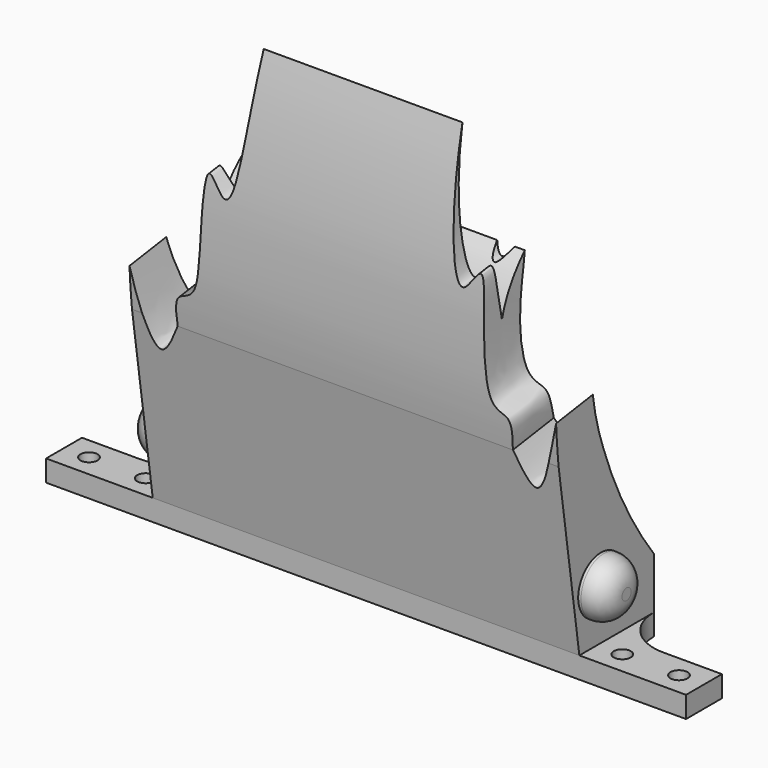
from build123d import *

# Parameters (mm, degrees)
F0_R      = 1.5
F1_DEPTH  = 3.75
F2_W      = 75
F2_H      = 7.89
F3_DEPTH  = 10
F4_W      = 75
F4_H      = 13.75
F5_DEPTH  = 25
F7_DEPTH  = 108.8
F9_DEPTH  = 25
F10_W     = 23.3560199849
F10_H     = 16.445
F11_DEPTH = 5
F15_DEPTH = 75
F17_DEPTH = 25
F19_R     = 8.4497474683
F20_DEPTH = 4
F22_DEPTH = 113.6
F23_R     = 5
F24_DEPTH = 4.5
F25_R     = 4
F26_R     = 5
F27_DEPTH = 4.5
F28_R     = 4


# Not quite as in the source:
# - a feature of the source that left no trace in its solid (it failed there, or was rolled back) is left out


with BuildPart() as f1:
    # F0 (on Top) → F1 (new body)
    with BuildSketch(Plane.XY):
        Polygon((-20.03, 3.5297368421), (-38.78, 3.5297368421), (-38.78, -4.3602631579), (73.72, -4.3602631579), (73.72, 3.5297368421), align=None)
        with Locations((-34.39, -0.4152631579)):
            Circle(F0_R, mode=Mode.SUBTRACT)
        with BuildLine():
            ThreePointArc((-22.92, -0.4152631579), (-24.42, -1.9152631579), (-25.92, -0.4152631579))
            ThreePointArc((-25.92, -0.4152631579), (-24.42, 1.0847368421), (-22.92, -0.4152631579))
        make_face(mode=Mode.SUBTRACT)
        with Locations((-15.64, -0.4152631579)):
            Circle(F0_R, mode=Mode.SUBTRACT)
        with Locations((-5.67, -0.4152631579)):
            Circle(F0_R, mode=Mode.SUBTRACT)
        with Locations((3.11, -0.4152631579)):
            Circle(F0_R, mode=Mode.SUBTRACT)
        with Locations((13.08, -0.4152631579)):
            Circle(F0_R, mode=Mode.SUBTRACT)
        with Locations((21.86, -0.4152631579)):
            Circle(F0_R, mode=Mode.SUBTRACT)
        with Locations((31.83, -0.4152631579)):
            Circle(F0_R, mode=Mode.SUBTRACT)
        with Locations((40.61, -0.4152631579)):
            Circle(F0_R, mode=Mode.SUBTRACT)
        with Locations((50.58, -0.4152631579)):
            Circle(F0_R, mode=Mode.SUBTRACT)
        with Locations((59.36, -0.4152631579)):
            Circle(F0_R, mode=Mode.SUBTRACT)
        with Locations((69.33, -0.4152631579)):
            Circle(F0_R, mode=Mode.SUBTRACT)
    extrude(amount=F1_DEPTH)

    # F2 (on face) → F3 (join)
    with BuildSketch(Plane.XY.offset(3.75)):
        with Locations((17.47, -0.4152631579)):
            Rectangle(F2_W, F2_H)
    extrude(amount=F3_DEPTH)

    # F4 (on face) → F5 (join)
    with BuildSketch(Plane(origin=(0, 3.5297368421, 0), x_dir=(-1, 0, 0), z_dir=(0, 1, 0))):
        with Locations((-17.47, 6.875)):
            Rectangle(F4_W, F4_H)
    extrude(amount=F5_DEPTH)

    # F6 (on face) → F7 (cut)
    with BuildSketch(Plane(origin=(-20.03, 0, 0), x_dir=(0, -1, 0), z_dir=(-1, 0, 0))):
        with BuildLine():
            Line((-28.5297368421, 13.75), (-28.5297368421, 1.3423696908))
            add(Edge.make_bspline(
                [(-28.5297368421, 1.3423696908), (-28.4407085002, 1.8407238057), (-27.4309487298, 4.2160851583), (-18.5019975598, 9.7006212436), (-25.1355636842, 11.5607893027), (-17.452811929, 12.8495323479), (-12.0847368421, 13.75)],
                knots=[0.0902573519, 0.0902573519, 0.0902573519, 0.0902573519, 0.1853961314, 0.5083170397, 0.656452384, 1, 1, 1, 1], degree=3))
            Line((-12.0847368421, 13.75), (-28.5297368421, 13.75))
        make_face()
    extrude(amount=-F7_DEPTH, mode=Mode.SUBTRACT)

    # F8 (on face) → F9 (cut)
    with BuildSketch(Plane.XY.offset(13.75)):
        with BuildLine():
            Line((-20.03, 28.5297368421), (-20.03, 12.0847368421))
            add(Edge.make_bspline(
                [(-20.03, 12.0847368421), (-16.6011347781, 15.620817943), (-11.1074776006, 21.8320831182), (-6.6512433884, 13.3190321336), (-3.164406946, 31.8472349575), (7.0542574353, 21.7542281947), (14.4432723922, 26.9517716178), (17.47, 28.5297368421)],
                knots=[0, 0, 0, 0, 0.2253636629, 0.3548505417, 0.5781774765, 0.7768820918, 1, 1, 1, 1], degree=3))
            Line((17.47, 28.5297368421), (-20.03, 28.5297368421))
        make_face()
        with BuildLine():
            Line((54.97, 28.5297368421), (17.47, 28.5297368421))
            add(Edge.make_bspline(
                [(54.97, 12.0847368421), (51.5411347781, 15.620817943), (46.0474776006, 21.8320831182), (41.5912433884, 13.3190321336), (38.104406946, 31.8472349575), (27.8857425647, 21.7542281947), (20.4967276078, 26.9517716178), (17.47, 28.5297368421)],
                knots=[0, 0, 0, 0, 0.2253636629, 0.3548505417, 0.5781774765, 0.7768820918, 1, 1, 1, 1], degree=3))
            Line((54.97, 12.0847368421), (54.97, 28.5297368421))
        make_face()
    extrude(amount=-F9_DEPTH, mode=Mode.SUBTRACT)

    # F10 (on face) → F11 (join)
    with BuildSketch(Plane.XY.offset(13.75)):
        with Locations((28.7449785974, 3.8622368421)):
            Rectangle(F10_W, F10_H)
        with Locations((5.3889586125, 3.8622368421)):
            Rectangle(F10_W, F10_H)
        Polygon((17.0669686049, 17.9865639657), (17.0669686049, 12.0847368421), (40.4229885899, 12.0847368421), align=None)
        Polygon((17.0669686049, 17.9865639657), (-6.28905138, 12.0847368421), (17.0669686049, 12.0847368421), align=None)
    extrude(amount=F11_DEPTH)

    # F14 (on face) → F15 (join)
    with BuildSketch(Plane(origin=(-20.03, 0, 0), x_dir=(0, -1, 0), z_dir=(-1, 0, 0))):
        with BuildLine():
            Line((4.3602631579, 0), (4.3602631579, 3.75))
            Line((4.3602631579, 3.75), (8.9196669428, 34.7869201625))
            ThreePointArc((8.9196669428, 34.7869201625), (9.1775200626, 57.5848380943), (5.009538897, 80))
            ThreePointArc((5.009538897, 80), (6.7748915404, 66.0775688262), (5.5820018111, 52.0944513684))
            ThreePointArc((5.5820018111, 52.0944513684), (3.0013036661, 42.5791343604), (-0.9565926029, 33.5493880847))
            ThreePointArc((-0.9565926029, 33.5493880847), (-8.0005792846, 22.8777948312), (-16.9551318954, 13.75))
            Line((-16.9551318954, 13.75), (-5.9577007778, 13.75))
            Line((-5.9577007778, 13.75), (-5.9577007778, 0))
            Line((-5.9577007778, 0), (4.3602631579, 0))
        make_face()
        with BuildLine():
            ThreePointArc((-0.9565926029, 33.5493880847), (3.0013036661, 42.5791343604), (5.5820018111, 52.0944513684))
            ThreePointArc((5.5820018111, 52.0944513684), (3.4443763791, 56.7010859278), (0, 60.4329481721))
            ThreePointArc((0, 60.4329481721), (1.7419135243, 46.9121668247), (-0.9565926029, 33.5493880847))
        make_face()
    extrude(amount=-F15_DEPTH)

    # F16 (on face) → F17 (cut)
    with BuildSketch(Plane(origin=(0, -3.7289072702, -0.5477861151), x_dir=(1, 0, 0), z_dir=(0, -0.9893813749, -0.145342681))):
        with BuildLine():
            Line((54.97, 79.8786098093), (34.94, 79.8786098093))
            add(Edge.make_bspline(
                [(34.94, 79.8786098093), (35.5747336463, 67.1946130241), (36.8101432908, 52.6348357258), (43.2912977366, 66.5575151279), (41.2646113617, 40.614999334), (47.2719465236, 41.4600702356), (47.0529437754, 37.7844129566), (46.9294752279, 35.7139392073)],
                knots=[0, 0, 0, 0, 0.3123634265, 0.4432138602, 0.7268454095, 0.853271119, 1, 1, 1, 1], degree=3))
            add(Edge.make_bspline(
                [(46.9294752279, 35.7139392073), (48.1657861662, 33.1189822824), (51.1577924939, 26.7936633153), (53.5903321083, 36.776473437), (54.97, 42.6643975079)],
                knots=[0, 0, 0, 0, 0.4103383117, 1, 1, 1, 1], degree=3))
            Line((54.97, 42.6643975079), (54.97, 79.8786098093))
        make_face()
        with BuildLine():
            add(Edge.make_bspline(
                [(0, 79.8786098093), (-0.6347336463, 67.1946130241), (-1.8701432908, 52.6348357258), (-8.3512977366, 66.5575151279), (-6.3246113617, 40.614999334), (-12.3319465236, 41.4600702356), (-12.1129437754, 37.7844129566), (-11.9894752279, 35.7139392073)],
                knots=[0, 0, 0, 0, 0.3123634265, 0.4432138602, 0.7268454095, 0.853271119, 1, 1, 1, 1], degree=3))
            Line((0, 79.8786098093), (-20.03, 79.8786098093))
            Line((-20.03, 79.8786098093), (-20.03, 42.6643975079))
            add(Edge.make_bspline(
                [(-11.9894752279, 35.7139392073), (-13.2257861662, 33.1189822824), (-16.2177924939, 26.7936633153), (-18.6503321083, 36.776473437), (-20.03, 42.6643975079)],
                knots=[0, 0, 0, 0, 0.4103383117, 1, 1, 1, 1], degree=3))
        make_face()
    extrude(amount=-F17_DEPTH, mode=Mode.SUBTRACT)

    # F19
    f19_edges = [f1.edges().sort_by_distance(p)[0] for p in [
        (54.97, 3.529737, 1.875),
        (-20.03, 3.529737, 1.875),
    ]]
    fillet(f19_edges, radius=F19_R)

    # F0 (on Top) → F20 (cut)
    with BuildSketch(Plane.XY):
        with Locations((-15.64, -0.4152631579)):
            Circle(F0_R)
        with Locations((-5.67, -0.4152631579)):
            Circle(F0_R)
        with Locations((3.11, -0.4152631579)):
            Circle(F0_R)
        with Locations((13.08, -0.4152631579)):
            Circle(F0_R)
        with Locations((21.86, -0.4152631579)):
            Circle(F0_R)
        with Locations((31.83, -0.4152631579)):
            Circle(F0_R)
        with Locations((50.58, -0.4152631579)):
            Circle(F0_R)
        with Locations((40.61, -0.4152631579)):
            Circle(F0_R)
    extrude(amount=F20_DEPTH, mode=Mode.SUBTRACT)

    # F21 (on face) → F22 (cut)
    with BuildSketch(Plane(origin=(-20.03, 0, 0), x_dir=(0, -1, 0), z_dir=(-1, 0, 0))):
        with BuildLine():
            Line((-34.5777980983, 0), (-24.266862789, 0))
            ThreePointArc((-24.266862789, 0), (-10.3134953642, 15.1778715767), (-0.9565926029, 33.5493880847))
            Line((-0.9565926029, 33.5493880847), (-34.5777980983, 33.5493880847))
            Line((-34.5777980983, 33.5493880847), (-34.5777980983, 0))
        make_face()
    extrude(amount=-F22_DEPTH, mode=Mode.SUBTRACT)

    # F23 (on face) → F24 (join)
    with BuildSketch(Plane.YZ.offset(54.97)):
        with Locations((0.3820091246, 12.75)):
            Circle(F23_R)
    extrude(amount=F24_DEPTH)

    # F25
    f25_edges = [f1.edges().sort_by_distance(p)[0] for p in [
        (59.47, -4.617991, 12.75),
    ]]
    fillet(f25_edges, radius=F25_R)

    # F26 (on face) → F27 (join)
    with BuildSketch(Plane(origin=(-20.03, 0, 0), x_dir=(0, -1, 0), z_dir=(-1, 0, 0))):
        with Locations((-0.3820091246, 12.75)):
            Circle(F26_R)
    extrude(amount=F27_DEPTH)

    # F28
    f28_edges = [f1.edges().sort_by_distance(p)[0] for p in [
        (-24.53, 5.382009, 12.75),
    ]]
    fillet(f28_edges, radius=F28_R)


solid = f1.part
